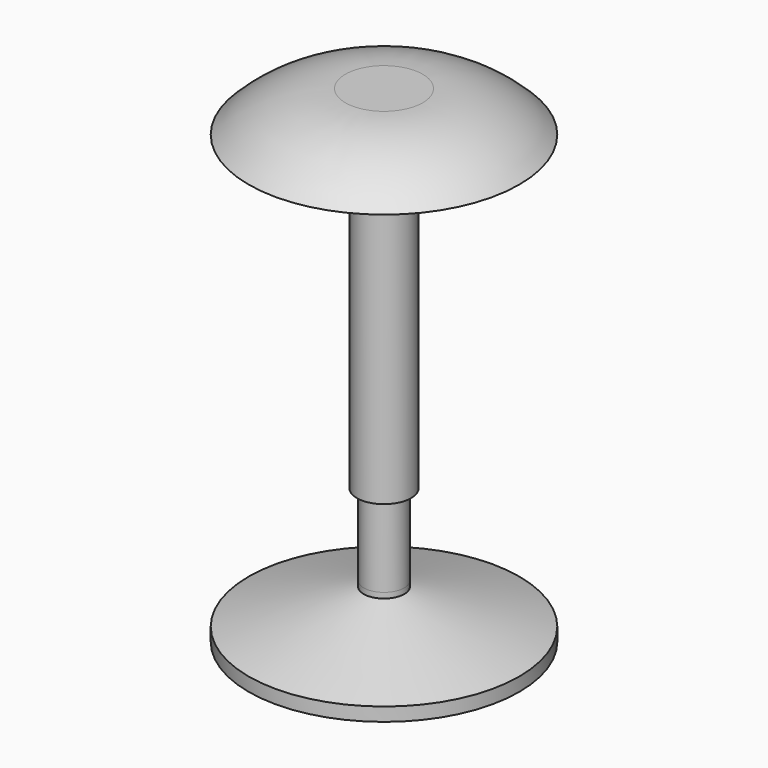
from build123d import *

# Parameters (mm, degrees)
F0_R        = 6.35
F1_DEPTH    = 2.54
F2_R        = 0.9525
F3_DEPTH    = 3.81
F4_R        = 1.27
F5_DEPTH    = 12.7
F6_R        = 6.35
F7_DEPTH    = 3.81
F8_S5_R     = 0.9525
F8_T6_DEPTH = 11
F9_S5_R     = 1.27
F9_T6_DEPTH = 11


# Not quite as in the source:
# - a fillet or chamfer that OpenCascade refuses, or shapes differently, is made with other operations: its cross-section is extruded or revolved along the edge and cut away or added


with BuildPart() as f1:
    # F0 (on Top) → F1 (new body)
    with BuildSketch(Plane.XY):
        Circle(F0_R)
    extrude(amount=F1_DEPTH)

    # F2 (on face) → F3 (join)
    with BuildSketch(Plane.XY.offset(2.54)):
        Circle(F2_R)
    extrude(amount=F3_DEPTH)

    # F4 (on face) → F5 (join)
    with BuildSketch(Plane.XY.offset(6.35)):
        Circle(F4_R)
    extrude(amount=F5_DEPTH)

    # F6 (on face) → F7 (join)
    with BuildSketch(Plane.XY.offset(19.05)):
        Circle(F6_R)
    extrude(amount=F7_DEPTH)

    # F8: chamfer of 1.905 x 6.2309742382 on 1 edges, made by hand


with BuildPart() as f8_tool2:
    # F8_s3 → F8_t4 (revolve)
    with BuildSketch(Plane.XZ):
        Polygon((0.1190257618, 2.54), (6.35, 0.635), (6.35, 2.54), align=None)
    revolve(axis=Axis((0, 0, 2.54), (0, 0, 1)))

    # F8_s5 → F8_t6 (cut, symmetric)
    with BuildSketch(Plane.XY.offset(1.6)):
        Circle(F8_S5_R)
    extrude(amount=F8_T6_DEPTH, both=True, mode=Mode.SUBTRACT)


with BuildPart() as f1_1:
    add(f1.part)

    # F8_t1: cut F8_tool2
    add(f8_tool2.part, mode=Mode.SUBTRACT)

    # F9: chamfer of 1.905 x 6.2309742382 on 1 edges, made by hand


with BuildPart() as f9_tool2:
    # F9_s3 → F9_t4 (revolve)
    with BuildSketch(Plane.XZ):
        Polygon((6.35, 20.955), (0.1190257618, 19.05), (6.35, 19.05), align=None)
    revolve(axis=Axis((0, 0, 19.05), (0, 0, 1)))

    # F9_s5 → F9_t6 (cut, symmetric)
    with BuildSketch(Plane.XY.offset(20)):
        Circle(F9_S5_R)
    extrude(amount=F9_T6_DEPTH, both=True, mode=Mode.SUBTRACT)


with BuildPart() as f1_2:
    add(f1_1.part)

    # F9_t1: cut F9_tool2
    add(f9_tool2.part, mode=Mode.SUBTRACT)

    # F10: fillet of radius 6.35 on 1 edges, made by hand

    # F10_s1 → F10_t2 (revolve, cut)
    with BuildSketch(Plane.XZ):
        with BuildLine():
            ThreePointArc((6.35, 20.955), (4.2745373727, 22.3644107304), (1.8151929479, 22.86))
            Line((1.8151929479, 22.86), (6.35, 22.86))
            Line((6.35, 22.86), (6.35, 20.955))
        make_face()
    revolve(axis=Axis((0, 0, 22.86), (0, 0, 1)), mode=Mode.SUBTRACT)


solid = f1_2.part
